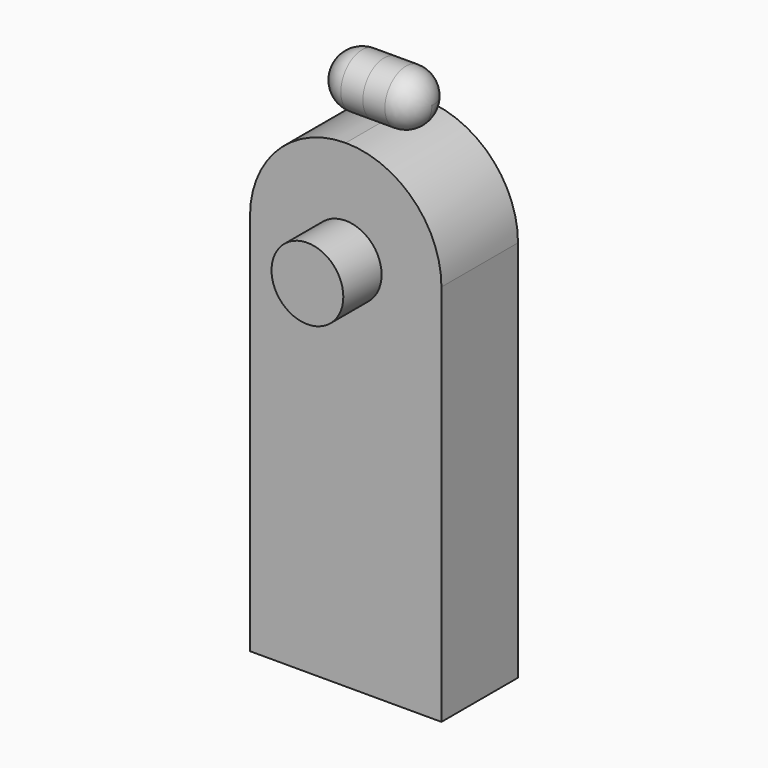
from build123d import *

# Parameters (mm, degrees)
F0_W     = 50.8
F0_H     = 127
F1_DEPTH = 12.7
F2_R     = 25.39999
F3_R     = 9.525
F4_DEPTH = 25.4
F6_DEPTH = 12.7
F7_R     = 6.858


# Not quite as in the source:
# - a fillet or chamfer is up to 0.001 mm smaller than in the source, because OpenCascade refuses the exact size


with BuildPart() as f1:
    # F0 (on Front) → F1 (new body, symmetric)
    with BuildSketch(Plane.XZ):
        Rectangle(F0_W, F0_H)
    extrude(amount=F1_DEPTH, both=True)

    # F2 (radius 25.4 in the source; OpenCascade refuses exactly that, so slightly less here)
    f2_edges = [f1.edges().sort_by_distance(p)[0] for p in [
        (-25.4, 0, 63.5),
        (25.4, 0, 63.5),
    ]]
    fillet(f2_edges, radius=F2_R)

    # F3 (on Front) → F4 (join, symmetric)
    with BuildSketch(Plane.XZ):
        with Locations((0, 35.8093136142)):
            Circle(F3_R)
    extrude(amount=F4_DEPTH, both=True)


with BuildPart() as f6:
    # F5 (on Right) → F6 (new body, symmetric)
    with BuildSketch(Plane.YZ):
        with BuildLine():
            ThreePointArc((0, 64.1574280324), (4.9593605279, 66.2116624237), (7.0135949192, 71.1710229516))
            ThreePointArc((7.0135949192, 71.1710229516), (-4.9593605279, 76.1303834795), (0, 64.1574280324))
        make_face()
    extrude(amount=F6_DEPTH, both=True)

    # F7
    f7_edges = [f6.edges().sort_by_distance(p)[0] for p in [
        (-12.7, -4.959361, 76.130383),
        (12.7, 4.959361, 66.211662),
        (12.7, -4.959361, 76.130383),
    ]]
    fillet(f7_edges, radius=F7_R)


solid = Compound([f1.part, f6.part])
